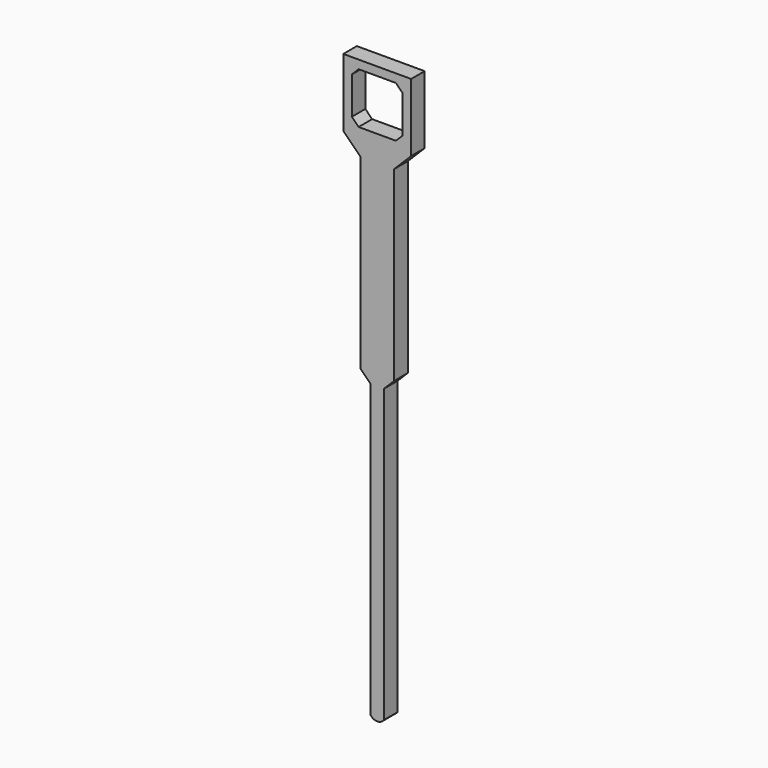
from build123d import *

# Parameters (mm, degrees)
F0_W        = 5.08
F0_H        = 114.3
F1_DEPTH    = 6.35
F2_SIZE     = 1.27
F3_R        = 2.54
F4_T1_DEPTH = 6.35
F4_T6_DEPTH = 6.35
F5_SIZE     = 2.54
F6_T1_DEPTH = 6.35
F6_T6_DEPTH = 6.35


# Not quite as in the source:
# - a fillet or chamfer that OpenCascade refuses, or shapes differently, is made with other operations: its cross-section is extruded or revolved along the edge and cut away or added


with BuildPart() as f1:
    # F0 (on Front) → F1 (new body)
    with BuildSketch(Plane.XZ):
        Polygon((12.7, 38.1), (12.7, 63.5), (-12.7, 63.5), (-12.7, 38.1), (-6.3373190351, 38.1), (-6.3373190351, -38.1), (-2.54, -38.1), (2.54, -38.1), (6.3626809649, -38.1), (6.3626809649, 38.1), align=None)
        Polygon((-9.5123190351, 60.325), (9.5376809649, 60.325), (9.5376809649, 41.275), (6.3626809649, 41.275), (-6.3373190351, 41.275), (-9.5123190351, 41.275), align=None, mode=Mode.SUBTRACT)
        with Locations((0, -95.25)):
            Rectangle(F0_W, F0_H)
    extrude(amount=F1_DEPTH)

    # F2
    f2_edges = [f1.edges().sort_by_distance(p)[0] for p in [
        (-2.54, -3.175, -152.4),
        (2.54, -3.175, -152.4),
    ]]
    chamfer(f2_edges, length=F2_SIZE)

    # F3
    f3_edges = [f1.edges().sort_by_distance(p)[0] for p in [
        (-1.27, -3.175, -152.4),
        (1.27, -3.175, -152.4),
    ]]
    fillet(f3_edges, radius=F3_R)

    # F4: chamfer of 3.81 on 2 edges, made by hand

    # F4_s2 → F4_t1 (join)
    with BuildSketch(Plane.XZ):
        Polygon((2.54, -41.91), (6.35, -38.1), (2.54, -38.1), align=None)
    extrude(amount=F4_T1_DEPTH)


with BuildPart() as f4_tool4:
    # F4_s5 → F4_t6 (new body)
    with BuildSketch(Plane.XZ):
        Polygon((-2.54, -41.91), (-6.35, -38.1), (-2.54, -38.1), align=None)
    extrude(amount=F4_T6_DEPTH)

    split(bisect_by=Plane.YZ.offset(-6.3373190351), keep=Keep.TOP)


with BuildPart() as f1_1:
    add(f1.part)

    # F4_t3: union F4_tool4
    add(f4_tool4.part)

    # F5
    f5_edges = [f1_1.edges().sort_by_distance(p)[0] for p in [
        (-9.512319, -3.175, 60.325),
        (9.537681, -3.175, 60.325),
        (-9.512319, -3.175, 41.275),
        (9.537681, -3.175, 41.275),
    ]]
    chamfer(f5_edges, length=F5_SIZE)

    # F6: chamfer of 6.35 on 2 edges, made by hand

    # F6_s2 → F6_t1 (join)
    with BuildSketch(Plane.XZ):
        Polygon((-12.6873190351, 38.1), (-6.3373190351, 31.75), (-6.3373190351, 38.1), align=None)
    extrude(amount=F6_T1_DEPTH)


with BuildPart() as f6_tool4:
    # F6_s5 → F6_t6 (new body)
    with BuildSketch(Plane.XZ):
        Polygon((6.3626809649, 31.75), (12.7126809649, 38.1), (6.3626809649, 38.1), align=None)
    extrude(amount=F6_T6_DEPTH)

    split(bisect_by=Plane.YZ.offset(12.7), keep=Keep.BOTTOM)


with BuildPart() as f1_2:
    add(f1_1.part)

    # F6_t3: union F6_tool4
    add(f6_tool4.part)


solid = f1_2.part
